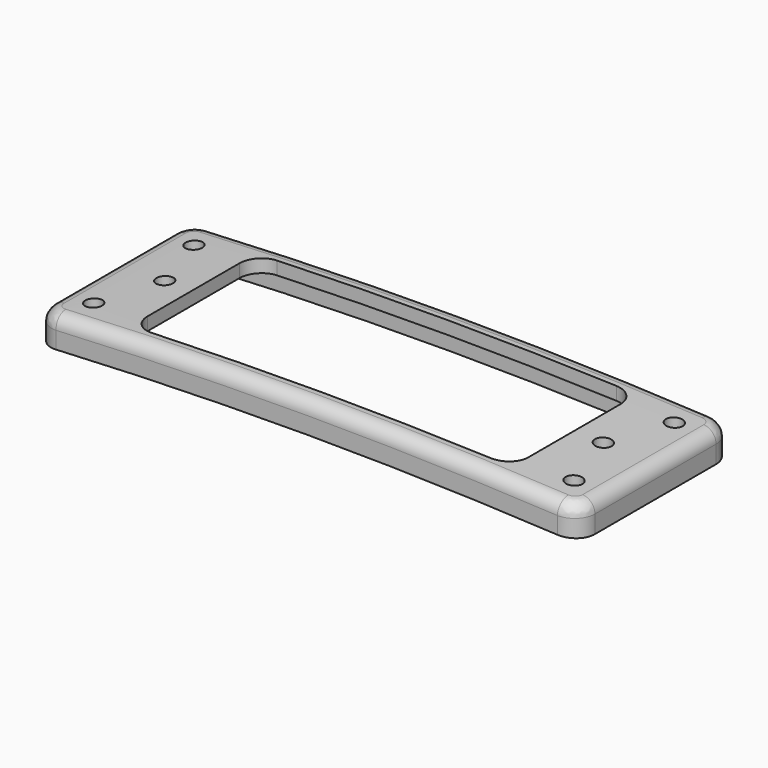
from build123d import *

# Parameters (mm, degrees)
F1_DEPTH = 18.5
F2_R     = 4
F3_R     = 2.5
F4_T     = 2.5
F6_DEPTH = 7.2510001
F7_R     = 1.6
F8_DEPTH = 7.2510001


# Not quite as in the source:
# - a shell that OpenCascade refuses in one call is made with other operations: the cavity is built on its own and cut out


with BuildPart() as f1:
    # F0 (on Front) → F1 (new body, symmetric)
    with BuildSketch(Plane.XZ):
        with BuildLine():
            ThreePointArc((-52, 0), (0, 1.5), (52, 0))
            Line((52, 0), (52, 5.7595163164))
            ThreePointArc((52, 5.7595163164), (0, 7.25), (-52, 5.7595163164))
            Line((-52, 5.7595163164), (-52, 0))
        make_face()
    extrude(amount=F1_DEPTH, both=True)

    # F2
    f2_edges = [f1.edges().sort_by_distance(p)[0] for p in [
        (-52, -18.5, 2.879758),
        (52, -18.5, 2.879758),
        (52, 18.5, 2.879758),
        (-52, 18.5, 2.879758),
    ]]
    fillet(f2_edges, radius=F2_R)

    # F3
    f3_edges = [f1.edges().sort_by_distance(p)[0] for p in [
        (0, 18.5, 7.25),
        (50.827405, 17.329449, 5.826031),
        (-50.827405, 17.329449, 5.826031),
        (52, 0, 5.759516),
        (-52, 0, 5.759516),
        (50.827405, -17.329449, 5.826031),
        (-50.827405, -17.329449, 5.826031),
        (0, -18.5, 7.25),
    ]]
    fillet(f3_edges, radius=F3_R)

    # F4: shell of thickness 2.5, made by hand


with BuildPart() as f4_core1:
    # F4_t2: copy of F1
    add(f1.part)

    # the walls: a layer under each face that stays
    f4_faces = [f4_core1.faces().sort_by_distance(p)[0] for p in [
        (-52, 0, 1.6978781362),
        (-50.8284271247, 17.3284271247, 1.7383225056),
        (-50.8284271247, -17.3284271247, 1.7383225056),
        (-50.5083309751, 16.6505657676, 5.1471783261),
        (0, 18.5, 2.4860254539),
        (0, 0, 7.25),
        (-50.5083309751, -16.6505657676, 5.1471783261),
        (0, -18.5, 2.4860254539),
        (50.8284271247, 17.3284271247, 1.7383225056),
        (50.8284271247, -17.3284271247, 1.7383225056),
        (52, 0, 1.6978781362),
        (50.5090360778, 16.6497513661, 5.1471500034),
        (50.5090431938, -16.6497516105, 5.1471497822),
    ]]
    thicken(f4_faces, amount=-F4_T, mode=Mode.SUBTRACT)


with BuildPart() as f1_1:
    add(f1.part)

    # what is left inside the walls is the cavity
    f4_cavity = [f4_core1.part.solids().sort_by_distance(p)[0] for p in [
        (0, 5.333333, 1.525),
    ]]
    add(f4_cavity, mode=Mode.SUBTRACT)

    # F5 (on Top) → F6 (cut, through all)
    with BuildSketch(Plane.XY):
        with BuildLine():
            ThreePointArc((36.5, 11), (35.3284271247, 13.8284271247), (32.5, 15))
            Line((32.5, 15), (-32.5, 15))
            ThreePointArc((-32.5, 15), (-35.3284271247, 13.8284271247), (-36.5, 11))
            Line((-36.5, 11), (-36.5, -11))
            ThreePointArc((-36.5, -11), (-35.3284271247, -13.8284271247), (-32.5, -15))
            Line((-32.5, -15), (32.5, -15))
            ThreePointArc((32.5, -15), (35.3284271247, -13.8284271247), (36.5, -11))
            Line((36.5, -11), (36.5, 11))
        make_face()
    extrude(amount=F6_DEPTH, mode=Mode.SUBTRACT)

    # F7 (on Top) → F8 (cut, through all)
    with BuildSketch(Plane.XY):
        with Locations((-46, 12)):
            Circle(F7_R)
        with Locations((-42, 0)):
            Circle(F7_R)
        with Locations((-46, -12)):
            Circle(F7_R)
        with Locations((46, -12)):
            Circle(F7_R)
        with Locations((42, 0)):
            Circle(F7_R)
        with Locations((46, 12)):
            Circle(F7_R)
    extrude(amount=F8_DEPTH, mode=Mode.SUBTRACT)


solid = f1_1.part
